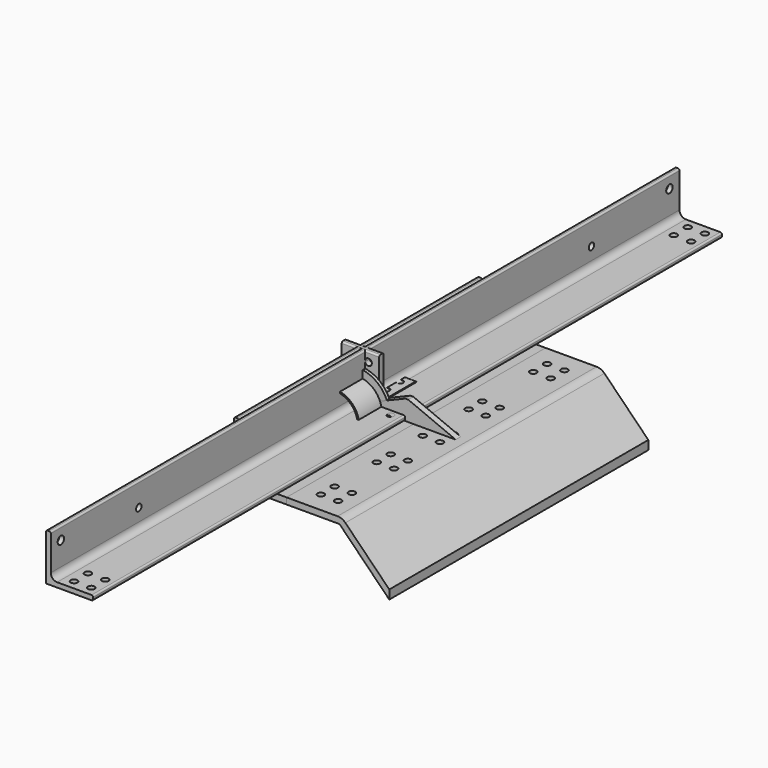
from build123d import *

# Parameters (mm, degrees)
F1_DEPTH  = 484
F3_D      = 21.5
F7_DEPTH  = 1250
F9_D      = 21.5
F11_D     = 21.5
F12_D     = 25.5
F14_DEPTH = 484
F16_D     = 21.5
F18_DEPTH = 59.5
F21_D     = 21.5
F22_D     = 21.5
F24_DEPTH = 515
F25_D     = 21.5
F27_R     = 76.2
F27_R_2   = 71.2
F28_DEPTH = 100
F29_R     = 100
F29_R_2   = 10.75
F30_DEPTH = 10
F33_DEPTH = 10
F34_DEPTH = 10


with BuildPart() as f1:
    # F0 (on Front) → F1 (new body, symmetric)
    with BuildSketch(Plane.XZ):
        with BuildLine():
            Line((0, 145), (0, 0))
            Line((0, 0), (145, 0))
            ThreePointArc((145, 0), (148.5355339059, 1.4644660941), (150, 5))
            Line((150, 5), (150, 10))
            ThreePointArc((150, 10), (148.5355339059, 13.5355339059), (145, 15))
            Line((145, 15), (35, 15))
            ThreePointArc((35, 15), (20.8578643763, 20.8578643763), (15, 35))
            Line((15, 35), (15, 145))
            ThreePointArc((15, 145), (13.5355339059, 148.5355339059), (10, 150))
            Line((10, 150), (5, 150))
            ThreePointArc((5, 150), (1.4644660941, 148.5355339059), (0, 145))
        make_face()
    extrude(amount=F1_DEPTH, both=True)

    # F3 (through all)
    with Locations(Plane(origin=(0, 0, 0), x_dir=(1, 0, 0), z_dir=(0, 0, -1))):
        with Locations((65, 450), (65, 395), (120, 395), (120, 450), (65, 227.5), (120, 227.5), (120, 172.5), (65, 172.5), (65, 45), (65, -10), (120, -10), (120, 45), (65, -137.5), (120, -137.5), (120, -192.5), (65, -192.5), (65, -395), (120, -395), (65, -450), (120, -450)):
            Hole(F3_D / 2)


with BuildPart() as f4_1:
    # F4: instance of F1
    add(f1.part.mirror(Plane.YZ))


with BuildPart() as f5_1:
    # F5: copy of F1
    add(f1.part.moved(Location((500, 0, 0))))


with BuildPart() as f7:
    # F0 (on Front) → F7 (new body, symmetric)
    with BuildSketch(Plane.XZ):
        with BuildLine():
            Line((0, 145), (0, 0))
            Line((0, 0), (145, 0))
            ThreePointArc((145, 0), (148.5355339059, 1.4644660941), (150, 5))
            Line((150, 5), (150, 10))
            ThreePointArc((150, 10), (148.5355339059, 13.5355339059), (145, 15))
            Line((145, 15), (35, 15))
            ThreePointArc((35, 15), (20.8578643763, 20.8578643763), (15, 35))
            Line((15, 35), (15, 145))
            ThreePointArc((15, 145), (13.5355339059, 148.5355339059), (10, 150))
            Line((10, 150), (5, 150))
            ThreePointArc((5, 150), (1.4644660941, 148.5355339059), (0, 145))
        make_face()
    extrude(amount=F7_DEPTH, both=True)

    # F9 (through all)
    with Locations(Plane(origin=(0, 0, 0), x_dir=(1, 0, 0), z_dir=(0, 0, -1))):
        with Locations((120, 1220), (65, 1220), (65, 1165), (120, 1165), (65, 30), (65, -30), (120, -30), (120, 30), (65, -1220), (120, -1220), (120, -1165), (65, -1165)):
            Hole(F9_D / 2)

    # F11 (through all)
    with Locations(Plane(origin=(0, 0, 0), x_dir=(0, 1, 0), z_dir=(-1, 0, 0))):
        with Locations((900, -75), (-900, -75)):
            Hole(F11_D / 2)

    # F12 (through all)
    with Locations(Plane(origin=(0, 0, 0), x_dir=(0, 1, 0), z_dir=(-1, 0, 0))):
        with Locations((-1210, -110), (1210, -110)):
            Hole(F12_D / 2)


with BuildPart() as f14:
    # F13 (on Front) → F14 (new body, symmetric)
    with BuildSketch(Plane.XZ):
        with BuildLine():
            ThreePointArc((3, 100), (0.8786796564, 99.1213203436), (0, 97))
            Line((0, 97), (0, 0))
            Line((0, 0), (97, 0))
            ThreePointArc((97, 0), (99.1213203436, 0.8786796564), (100, 3))
            Line((100, 3), (100, 7))
            ThreePointArc((100, 7), (99.1213203436, 9.1213203436), (97, 10))
            Line((97, 10), (22, 10))
            ThreePointArc((22, 10), (13.5147186258, 13.5147186258), (10, 22))
            Line((10, 22), (10, 97))
            ThreePointArc((10, 97), (9.1213203436, 99.1213203436), (7, 100))
            Line((7, 100), (3, 100))
        make_face()
    extrude(amount=F14_DEPTH, both=True)

    # F16 (through all)
    with Locations(Plane(origin=(0, 0, 0), x_dir=(1, 0, 0), z_dir=(0, 0, -1))):
        with Locations((72.5, -450), (72.5, -395), (72.5, 395), (72.5, 450)):
            Hole(F16_D / 2)


with BuildPart() as f18:
    # F17 (on Right) → F18 (new body, symmetric)
    with BuildSketch(Plane.YZ):
        with BuildLine():
            Line((0, 145), (0, 0))
            Line((0, 0), (145, 0))
            ThreePointArc((145, 0), (148.5355339059, 1.4644660941), (150, 5))
            Line((150, 5), (150, 13))
            ThreePointArc((150, 13), (148.5355339059, 16.5355339059), (145, 18))
            Line((145, 18), (38, 18))
            ThreePointArc((38, 18), (23.8578643763, 23.8578643763), (18, 38))
            Line((18, 38), (18, 145))
            ThreePointArc((18, 145), (16.5355339059, 148.5355339059), (13, 150))
            Line((13, 150), (5, 150))
            ThreePointArc((5, 150), (1.4644660941, 148.5355339059), (0, 145))
        make_face()
    extrude(amount=F18_DEPTH, both=True)

    # F21 (through all)
    with Locations(Plane(origin=(0, 0, 0), x_dir=(1, 0, 0), z_dir=(0, 0, -1))):
        with Locations((-25.5, -120), (29.5, -120), (29.5, -65), (-25.5, -65)):
            Hole(F21_D / 2)

    # F22 (through all)
    with Locations(Plane.XZ):
        with Locations((-29.5, 65), (25.5, 65), (25.5, 120), (-29.5, 120)):
            Hole(F22_D / 2)


with BuildPart() as f24:
    # F23 (on Front) → F24 (new body, symmetric)
    with BuildSketch(Plane.XZ):
        with BuildLine():
            Line((177, -20), (177, 0))
            Line((177, 0), (14.7669197382, 0))
            ThreePointArc((14.7669197382, 0), (1.2901934421, -2.6986401472), (-10.1083137321, -10.3784086664))
            Line((-10.1083137321, -10.3784086664), (-149.8599067098, -151.5696686491))
            Line((-149.8599067098, -151.5696686491), (-149.8599067098, -180))
            Line((-149.8599067098, -180), (-110.0206546917, -139.7503393747))
            Line((-110.0206546917, -139.7503393747), (5.0785333399, -23.4654439047))
            Line((5.0785333399, -23.4654439047), (5.5736174601, -22.965259619))
            ThreePointArc((5.5736174601, -22.965259619), (8.8303337955, -20.7710400421), (12.680827023, -20))
            Line((12.680827023, -20), (13.3845973021, -20))
            Line((13.3845973021, -20), (177, -20))
        make_face()
    extrude(amount=F24_DEPTH, both=True)

    # F25 (through all)
    with Locations(Plane.XY):
        with Locations((65, 450), (120, 450), (65, 395), (120, 395), (65, 192.5), (120, 192.5), (120, 137.5), (65, 137.5), (65, 10), (120, 10), (120, -45), (65, -45), (65, -172.5), (120, -172.5), (120, -227.5), (65, -227.5), (65, -395), (120, -450), (65, -450), (120, -395)):
            Hole(F25_D / 2)


with BuildPart() as f26_1:
    # F26: instance of F24
    add(f24.part.mirror(Plane(origin=(177, 0, -10), x_dir=(0, 1, 0), z_dir=(1, 0, 0))))


with BuildPart() as f28:
    # F27 (on Front) → F28 (new body)
    with BuildSketch(Plane.XZ):
        Circle(F27_R)
        Circle(F27_R_2, mode=Mode.SUBTRACT)
    extrude(amount=F28_DEPTH)


with BuildPart() as f30:
    # F29 (on Front) → F30 (new body)
    with BuildSketch(Plane.XZ):
        Circle(F29_R)
        Circle(F29_R_2, mode=Mode.SUBTRACT)
    extrude(amount=F30_DEPTH)


with BuildPart() as f33:
    # F32 (on face) → F33 (new body, symmetric)
    with BuildSketch(Plane.XZ):
        Polygon((160, 63), (151, 63), (0, 0), (311, 0), align=None)
    extrude(amount=F33_DEPTH, both=True)


with BuildPart() as f34:
    # F23 (on Front) → F34 (new body, symmetric)
    with BuildSketch(Plane.XZ):
        Polygon((117.0793650794, -45), (177, -20), (13.3845973021, -20), (9.231565321, -21.7327219524), (5.0785333399, -23.4654439047), (-110.0206546917, -139.7503393747), align=None)
    extrude(amount=F34_DEPTH, both=True)


solid = Compound([f1.part, f4_1.part, f7.part, f14.part, f18.part, f24.part, f26_1.part, f28.part, f30.part, f33.part, f34.part])
